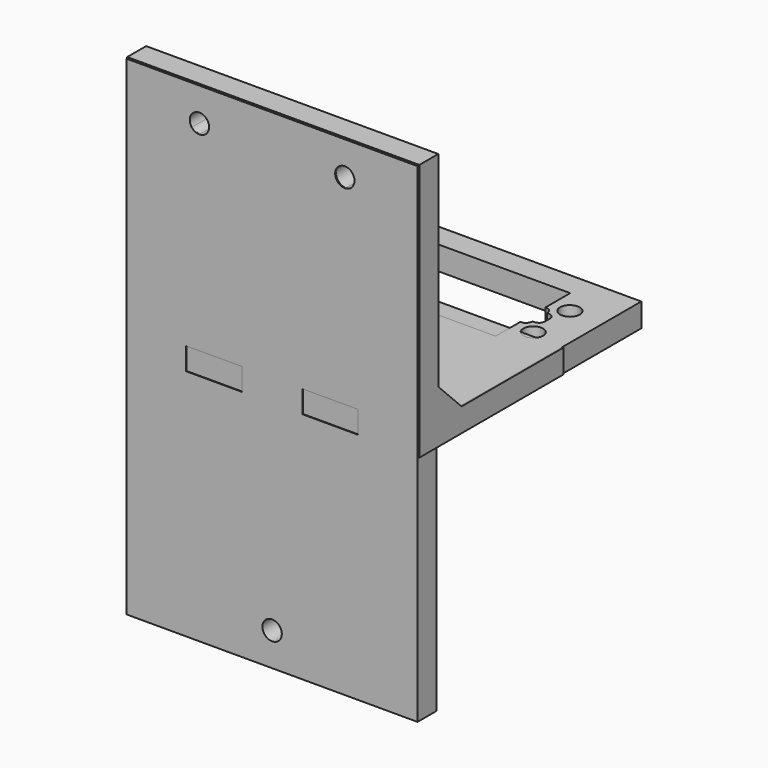
from build123d import *

# Parameters (mm, degrees)
F1_W      = 63.6524
F1_H      = 39.2176
F1_R      = 2.286
F1_W_2    = 40.64
F1_H_2    = 20.32
F2_DEPTH  = 2.5781
F3_W      = 63.6524
F3_H      = 56.1594
F3_R      = 2.2479
F4_DEPTH  = 5.1562
F5_SIZE   = 6.35
F6_R      = 2.1463
F7_DEPTH  = 2.5781
F8_W      = 63.373
F8_H      = 61.0362
F8_W_2    = 12.4206
F8_H_2    = 4.8768
F8_R      = 2.1082
F9_DEPTH  = 5.1562
F10_R     = 1.27
F11_W     = 63.373
F11_H     = 106.6038
F11_R     = 2.1082
F11_W_2   = 12.1412
F11_H_2   = 4.8768
F12_DEPTH = 5.1562


# Not quite as in the source:
# - a variable given as a bare number and used for a length is read in inches; the dataset says mm whatever the document's units were


with BuildPart() as f2:
    # F1 (on Top) → F2 (new body, symmetric)
    with BuildSketch(Plane.XY):
        with Locations((31.8262, 19.6088)):
            Rectangle(F1_W, F1_H)
        with Locations((7.4422, 18.8976)):
            Circle(F1_R, mode=Mode.SUBTRACT)
        with Locations((56.2102, 18.8976)):
            Circle(F1_R, mode=Mode.SUBTRACT)
        with Locations((7.4422, 28.9052)):
            Circle(F1_R, mode=Mode.SUBTRACT)
        with Locations((31.8262, 23.9014)):
            Rectangle(F1_W_2, F1_H_2, mode=Mode.SUBTRACT)
        with Locations((56.2102, 28.9052)):
            Circle(F1_R, mode=Mode.SUBTRACT)
    extrude(amount=F2_DEPTH, both=True)

    # F3 (on Front) → F4 (join)
    with BuildSketch(Plane.XZ):
        with Locations((31.8262, 25.5016)):
            Rectangle(F3_W, F3_H)
        with Locations((15.9131, 46.1772)):
            Circle(F3_R, mode=Mode.SUBTRACT)
        with Locations((47.7393, 46.1772)):
            Circle(F3_R, mode=Mode.SUBTRACT)
    extrude(amount=-F4_DEPTH)

    # F5
    f5_edges = [f2.edges().sort_by_distance(p)[0] for p in [
        (31.8262, 5.1562, 2.5781),
    ]]
    chamfer(f5_edges, length=F5_SIZE)


with BuildPart() as f7:
    # F6 (on Top) → F7 (new body, symmetric)
    with BuildSketch(Plane.XY):
        Polygon((63.373, 60.8076), (0, 60.8076), (0, 5.0165), (12.6576666667, 5.0165), (12.6576666667, 0), (25.3576666667, 0), (25.3576666667, 5.0165), (38.0153333333, 5.0165), (38.0153333333, 0), (50.7153333333, 0), (50.7153333333, 5.0165), (63.373, 5.0165), align=None)
        with Locations((7.3025, 40.4876)):
            Circle(F6_R, mode=Mode.SUBTRACT)
        with Locations((7.3025, 50.4952)):
            Circle(F6_R, mode=Mode.SUBTRACT)
        with BuildLine():
            Line((11.3665, 35.3314), (11.3665, 55.6514))
            Line((11.3665, 55.6514), (52.0065, 55.6514))
            Line((52.0065, 55.6514), (52.0065, 48.9204))
            Line((52.0065, 48.9204), (52.07, 48.9204))
            ThreePointArc((52.07, 48.9204), (53.1027294539, 48.4926294539), (53.5305, 47.4599))
            Line((53.5305, 47.4599), (55.1815, 47.4599))
            Line((55.1815, 47.4599), (55.1815, 43.5229))
            Line((55.1815, 43.5229), (53.5305, 43.5229))
            ThreePointArc((53.5305, 43.5229), (53.1027294539, 42.4901705461), (52.07, 42.0624))
            Line((52.07, 42.0624), (52.0065, 42.0624))
            Line((52.0065, 42.0624), (52.0065, 35.3314))
            Line((52.0065, 35.3314), (11.3665, 35.3314))
        make_face(mode=Mode.SUBTRACT)
        with Locations((56.0705, 40.4876)):
            Circle(F6_R, mode=Mode.SUBTRACT)
        with Locations((56.0705, 50.4952)):
            Circle(F6_R, mode=Mode.SUBTRACT)
    extrude(amount=F7_DEPTH, both=True)

    # F10
    f10_edges = [f7.edges().sort_by_distance(p)[0] for p in [
        (55.1815, 47.4599, 0),
        (55.1815, 43.5229, 0),
    ]]
    fillet(f10_edges, radius=F10_R)


with BuildPart() as f9:
    # F8 (on face) → F9 (new body)
    with BuildSketch(Plane.XZ.offset(-5.0165)):
        with Locations((31.6865, 22.7838)):
            Rectangle(F8_W, F8_H)
        with Locations((19.0076666667, 0)):
            Rectangle(F8_W_2, F8_H_2, mode=Mode.SUBTRACT)
        with Locations((44.3653333333, 0)):
            Rectangle(F8_W_2, F8_H_2, mode=Mode.SUBTRACT)
        with Locations((15.84325, 46.0375)):
            Circle(F8_R, mode=Mode.SUBTRACT)
        with Locations((47.52975, 46.0375)):
            Circle(F8_R, mode=Mode.SUBTRACT)
    extrude(amount=F9_DEPTH)


with BuildPart() as f12:
    # F11 (on face) → F12 (new body)
    with BuildSketch(Plane.XZ.offset(-5.0165)):
        with Locations((31.6865, 0)):
            Rectangle(F11_W, F11_H)
        with Locations((31.6865, -46.0375)):
            Circle(F11_R, mode=Mode.SUBTRACT)
        with Locations((19.0076666667, 0)):
            Rectangle(F11_W_2, F11_H_2, mode=Mode.SUBTRACT)
        with Locations((15.84325, 46.0375)):
            Circle(F11_R, mode=Mode.SUBTRACT)
        with Locations((44.3653333333, 0)):
            Rectangle(F11_W_2, F11_H_2, mode=Mode.SUBTRACT)
        with Locations((47.52975, 46.0375)):
            Circle(F11_R, mode=Mode.SUBTRACT)
    extrude(amount=F12_DEPTH)


solid = Compound([f2.part, f7.part, f9.part, f12.part])
